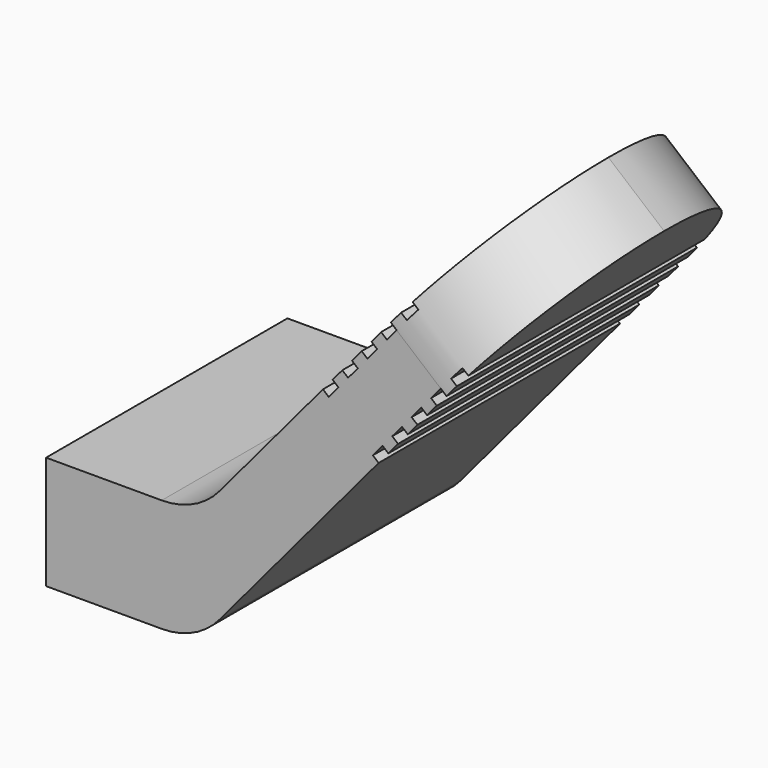
from build123d import *

# Parameters (mm, degrees)
F0_W     = 10
F0_H     = 7.5
F1_DEPTH = 20
F2_R     = 5
F3_R     = 9.99999
F4_R     = 5


# Not quite as in the source:
# - a fillet or chamfer is up to 0.001 mm smaller than in the source, because OpenCascade refuses the exact size


with BuildPart() as f1:
    # F0 (on Front) → F1 (new body)
    with BuildSketch(Plane.XZ):
        with Locations((5, 3.75)):
            Rectangle(F0_W, F0_H)
        Polygon((10, 7.5), (10, 0), (22.0492679997, 14.3597584268), (21.6662457782, 14.6811522316), (22.3090333878, 15.4471966748), (22.6920556094, 15.1258028699), (23.3348432191, 15.891847313), (22.9518209975, 16.2132411179), (23.5946086072, 16.979285561), (23.9776308288, 16.6578917562), (24.6204184385, 17.4239361993), (24.2373962169, 17.7453300041), (24.8801838266, 18.5113744472), (25.2632060482, 18.1899806424), (25.9059936578, 18.9560250855), (25.5229714363, 19.2774188904), (26.165759046, 20.0434633335), (26.5487812675, 19.7220695286), (27.1915688772, 20.4881139717), (26.8085466557, 20.8095077766), (27.4513342653, 21.5755522197), (27.8343564869, 21.2541584149), (32.9766573644, 27.3825139598), (29.2836282906, 30.4813332936), (24.1413274131, 24.3529777486), (24.5243496347, 24.0315839438), (23.881562025, 23.2655395007), (23.4985398034, 23.5869333055), (22.8557521937, 22.8208888624), (23.2387744153, 22.4994950575), (22.5959868056, 21.7334506144), (22.212964584, 22.0548444193), (21.5701769744, 21.2887999761), (21.9531991959, 20.9674061713), (21.3104115862, 20.2013617282), (20.9273893647, 20.522755533), (20.284601755, 19.7567110899), (20.6676239765, 19.4353172851), (20.0248363669, 18.6692728419), (19.6418141453, 18.9906666468), (18.9990265356, 18.2246222037), (19.3820487572, 17.9032283988), (18.7392611475, 17.1371839557), (18.3562389259, 17.4585777605), align=None)
    extrude(amount=F1_DEPTH)

    # F2
    f2_edges = [f1.edges().sort_by_distance(p)[0] for p in [
        (10, -10, 7.5),
    ]]
    fillet(f2_edges, radius=F2_R)

    # F3 (radius 10 in the source; OpenCascade refuses exactly that, so slightly less here)
    f3_edges = [f1.edges().sort_by_distance(p)[0] for p in [
        (31.130143, -20, 28.931924),
        (31.130143, 0, 28.931924),
    ]]
    fillet(f3_edges, radius=F3_R)

    # F4
    f4_edges = [f1.edges().sort_by_distance(p)[0] for p in [
        (10, -10, 0),
    ]]
    fillet(f4_edges, radius=F4_R)


solid = f1.part
